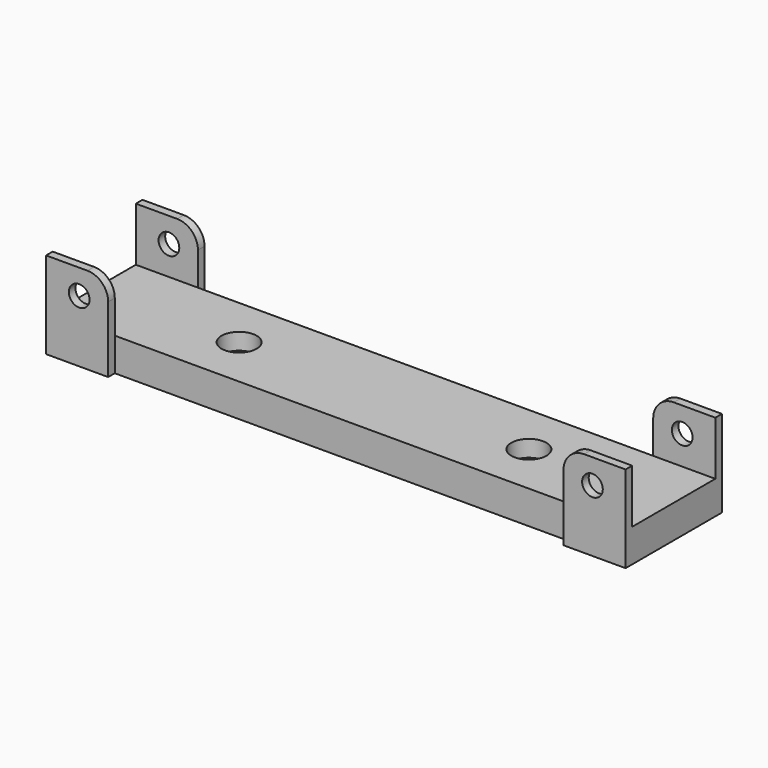
from build123d import *

# Parameters (mm, degrees)
F0_R     = 4.25
F0_R_2   = 2.25
F1_DEPTH = 8
F0_W     = 15
F0_H     = 2
F2_DEPTH = 21
F3_R     = 2.5
F4_DEPTH = 29.101
F5_R     = 5
F6_R     = 4.25
F7_DEPTH = 4


# Not quite as in the source:
# - a feature names something its author has since deleted; it is built from what else it names


with BuildPart() as f1:
    # F0 (on Top) → F1 (new body)
    with BuildSketch(Plane.XY):
        Polygon((55, -12.55), (70, -12.55), (70, 12.55), (55, 12.55), (-55, 12.55), (-70, 12.55), (-70, -12.55), (-55, -12.55), align=None)
        with Locations((-35, 0)):
            Circle(F0_R, mode=Mode.SUBTRACT)
        with Locations((35, 0)):
            Circle(F0_R, mode=Mode.SUBTRACT)
        with Locations((-35, 0)):
            Circle(F0_R)
        with Locations((-35, 0)):
            Circle(F0_R_2, mode=Mode.SUBTRACT)
        with Locations((35, 0)):
            Circle(F0_R)
        with Locations((35, 0)):
            Circle(F0_R_2, mode=Mode.SUBTRACT)
    extrude(amount=F1_DEPTH)

    # F0 (on Top) → F2 (join)
    with BuildSketch(Plane.XY):
        with Locations((-62.5, -13.55)):
            Rectangle(F0_W, F0_H)
        with Locations((62.5, -13.55)):
            Rectangle(F0_W, F0_H)
        with Locations((-62.5, 13.55)):
            Rectangle(F0_W, F0_H)
        with Locations((62.5, 13.55)):
            Rectangle(F0_W, F0_H)
    extrude(amount=F2_DEPTH)

    # F3 (on face) → F4 (cut, through all)
    with BuildSketch(Plane.XZ.offset(14.55)):
        with Locations((-62, 15)):
            Circle(F3_R)
        with Locations((62, 15)):
            Circle(F3_R)
    extrude(amount=-F4_DEPTH, mode=Mode.SUBTRACT)

    # F5
    f5_edges = [f1.edges().sort_by_distance(p)[0] for p in [
        (-55, -13.55, 21),
        (55, -13.55, 21),
        (-55, 13.55, 21),
        (55, 13.55, 21),
    ]]
    fillet(f5_edges, radius=F5_R)

    # F6 (on face) → F7 (cut)
    with BuildSketch(Plane.XY.offset(8)):
        with Locations((-35, 0)):
            Circle(F6_R)
        with Locations((35, 0)):
            Circle(F6_R)
    extrude(amount=-F7_DEPTH, mode=Mode.SUBTRACT)


solid = f1.part
